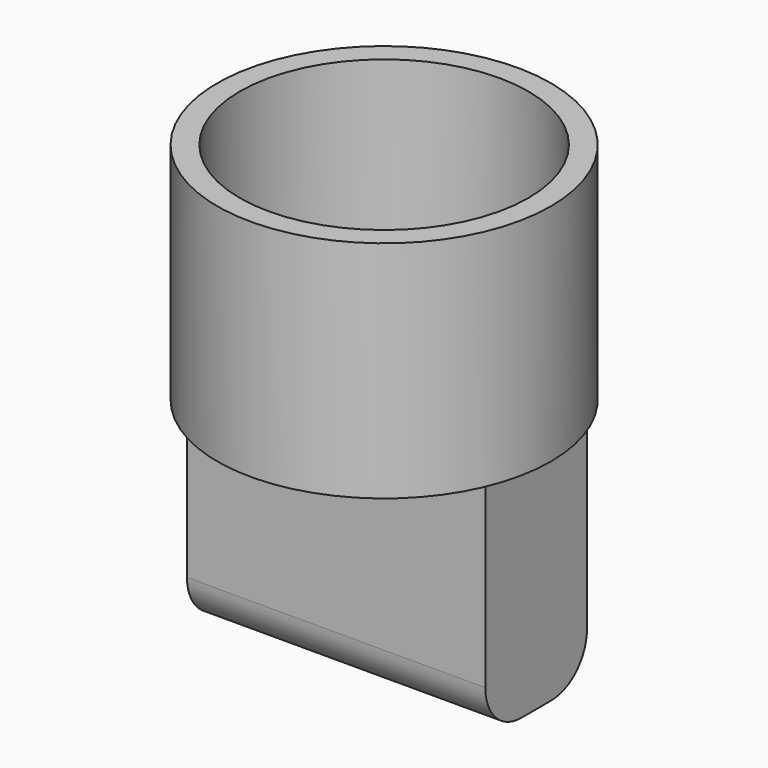
from build123d import *

# Parameters (mm, degrees)
F0_R         = 18.561525572
F1_DEPTH     = 25
F2_T         = -2.5
F3_W         = 33.1976041198
F3_H         = 14.1467070207
F4_DEPTH     = 25
F5_T         = -2.5
F7_DEPTH     = 3
F9_DEPTH     = 3
F10_T1_DEPTH = 58.1976041198
F11_T1_DEPTH = 58.1976041198


# Not quite as in the source:
# - a fillet or chamfer that OpenCascade refuses, or shapes differently, is made with other operations: its cross-section is extruded or revolved along the edge and cut away or added
# - a shell that OpenCascade refuses in one call is made with other operations: the cavity is built on its own and cut out


with BuildPart() as f1:
    # F0 (on Top) → F1 (new body)
    with BuildSketch(Plane.XY):
        Circle(F0_R)
    extrude(amount=F1_DEPTH)

    # F2
    f2_openings = [f1.faces().sort_by_distance(p)[0] for p in [
        (0, 0, 25),
        (0, 0, 0),
    ]]
    offset(amount=F2_T, openings=f2_openings)

    # F3 (on Top) → F4 (join)
    with BuildSketch(Plane.XY):
        with Locations((0.0943113118, 0.2829344012)):
            Rectangle(F3_W, F3_H)
    extrude(amount=-F4_DEPTH)

    # F5: a shell. OpenCascade refuses it in one call, so the cavity is built on its own and cut out:
    # the body offset inwards by the wall thickness, plus a prism from it out through each open face.
    f5_core = offset(f1.part, amount=F5_T, mode=Mode.PRIVATE)
    f5_exits = [f5_core.faces().sort_by_distance(p)[0] for p in [
        (0.094311, 0.282934, -22.5),
        (0.094311, 0.282934, -2.5),
    ]]
    add(f5_core, mode=Mode.SUBTRACT)
    extrude(f5_exits, amount=-F5_T, mode=Mode.SUBTRACT)

    # F6 (on Top) → F7 (join)
    with BuildSketch(Plane.XY):
        with BuildLine():
            Line((16.6573040187, -6.7166290246), (-16.5601819754, -6.760219112))
            ThreePointArc((-16.5601819754, -6.760219112), (0.0631717454, -17.8724120589), (16.6573040187, -6.7166290246))
        make_face()
    extrude(amount=F7_DEPTH)

    # F8 (on Top) → F9 (join)
    with BuildSketch(Plane.XY):
        with BuildLine():
            Line((-16.4011158049, 7.3119108565), (16.5623016655, 7.2848270647))
            ThreePointArc((16.5623016655, 7.2848270647), (0.0891507264, 17.7139786602), (-16.4011158049, 7.3119108565))
        make_face()
    extrude(amount=F9_DEPTH)

    # F10: fillet of radius 5 on 1 edges, made by hand

    # F10_s2 → F10_t1 (cut)
    with BuildSketch(Plane.YZ.offset(-29.004490748)):
        with BuildLine():
            ThreePointArc((-1.7904191092, -25), (-5.3259530151, -23.5355339059), (-6.7904191092, -20))
            Line((-6.7904191092, -20), (-6.7904191092, -25))
            Line((-6.7904191092, -25), (-1.7904191092, -25))
        make_face()
    extrude(amount=F10_T1_DEPTH, mode=Mode.SUBTRACT)

    # F11: fillet of radius 5 on 1 edges, made by hand

    # F11_s2 → F11_t1 (cut)
    with BuildSketch(Plane.YZ.offset(-29.004490748)):
        with BuildLine():
            ThreePointArc((7.3562879115, -20), (5.8918218175, -23.5355339059), (2.3562879115, -25))
            Line((2.3562879115, -25), (7.3562879115, -25))
            Line((7.3562879115, -25), (7.3562879115, -20))
        make_face()
    extrude(amount=F11_T1_DEPTH, mode=Mode.SUBTRACT)


solid = f1.part
